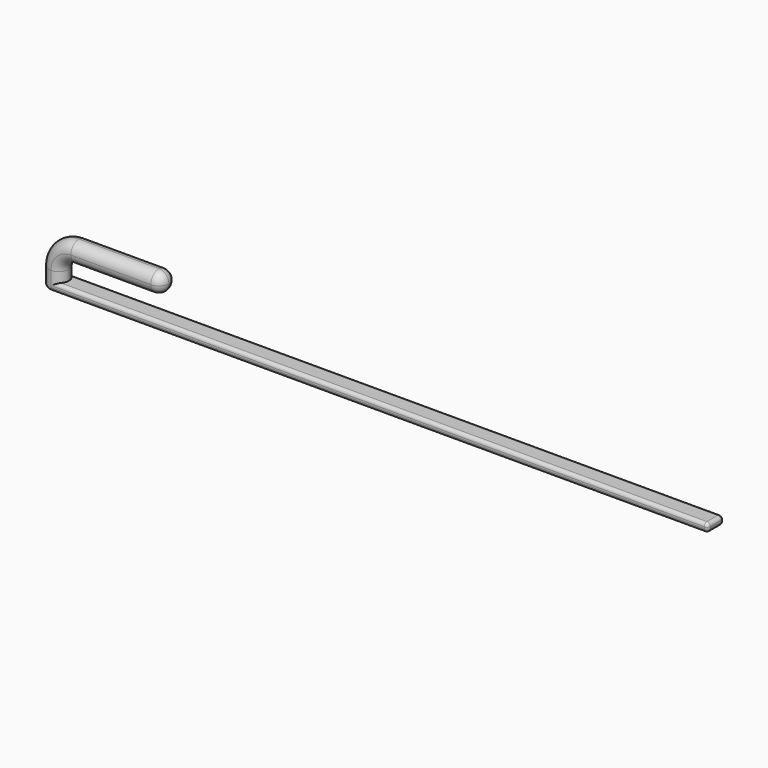
from build123d import *

# Parameters (mm, degrees)
F1_DEPTH = 7.62
F2_R     = 3.80999
F3_R     = 3.80999
F4_R     = 1.27
F5_R     = 1.27


# Not quite as in the source:
# - a fillet or chamfer is up to 0.001 mm smaller than in the source, because OpenCascade refuses the exact size


with BuildPart() as f1:
    # F0 (on Front) → F1 (new body)
    with BuildSketch(Plane.XZ):
        with BuildLine():
            Line((134.7724028379, 37.2032584392), (-111.6075971621, 37.2032584392))
            Line((-111.6075971621, 37.2032584392), (-111.6075971621, 41.0132584392))
            ThreePointArc((-111.6075971621, 41.0132584392), (-110.4916739984, 43.7073352756), (-107.7975971621, 44.8232584392))
            Line((-107.7975971621, 44.8232584392), (-73.5075971621, 44.8232584392))
            Line((-73.5075971621, 44.8232584392), (-73.5075971621, 52.4432584392))
            Line((-73.5075971621, 52.4432584392), (-107.7975971621, 52.4432584392))
            ThreePointArc((-107.7975971621, 52.4432584392), (-115.8798276711, 49.0954889482), (-119.2275971621, 41.0132584392))
            Line((-119.2275971621, 41.0132584392), (-119.2275971621, 39.1082584392))
            Line((-119.2275971621, 39.1082584392), (-119.2275971621, 37.2032584392))
            Line((-119.2275971621, 37.2032584392), (-119.2275971621, 34.0282584392))
            Line((-119.2275971621, 34.0282584392), (134.7724028379, 34.0282584392))
            Line((134.7724028379, 34.0282584392), (134.7724028379, 37.2032584392))
        make_face()
    extrude(amount=F1_DEPTH)

    # F2 (radius 3.81 in the source; OpenCascade refuses exactly that, so slightly less here)
    f2_edges = [f1.edges().sort_by_distance(p)[0] for p in [
        (-90.652597, -7.62, 52.443258),
        (-90.652597, -7.62, 44.823258),
        (-90.652597, 0, 44.823258),
        (-90.652597, 0, 52.443258),
    ]]
    fillet(f2_edges, radius=F2_R)

    # F3 (radius 3.81 in the source; OpenCascade refuses exactly that, so slightly less here)
    f3_edges = [f1.edges().sort_by_distance(p)[0] for p in [
        (-73.507597, -3.81, 52.443258),
        (-73.507597, -1.11592, 51.327338),
        (-73.507597, 0, 48.633258),
        (-73.507597, -1.11592, 45.939179),
        (-73.507597, -3.81, 44.823258),
        (-73.507597, -6.50408, 45.939179),
        (-73.507597, -6.50408, 51.327338),
        (-73.507597, -7.62, 48.633258),
    ]]
    fillet(f3_edges, radius=F3_R)

    # F4
    f4_edges = [f1.edges().sort_by_distance(p)[0] for p in [
        (11.582403, -7.62, 37.203258),
        (9.677398, -7.62, 34.028258),
        (11.582403, 0, 37.203258),
        (9.677398, 0, 34.028258),
    ]]
    fillet(f4_edges, radius=F4_R)

    # F5
    f5_edges = [f1.edges().sort_by_distance(p)[0] for p in [
        (134.772403, -7.248026, 36.831284),
        (134.772403, -7.62, 35.615758),
        (134.772403, -7.248026, 34.400233),
        (134.772403, -3.81, 34.028258),
        (134.772403, -0.371974, 34.400233),
        (134.772403, 0, 35.615758),
        (134.772403, -3.81, 37.203258),
        (134.772403, -0.371974, 36.831284),
    ]]
    fillet(f5_edges, radius=F5_R)


solid = f1.part
